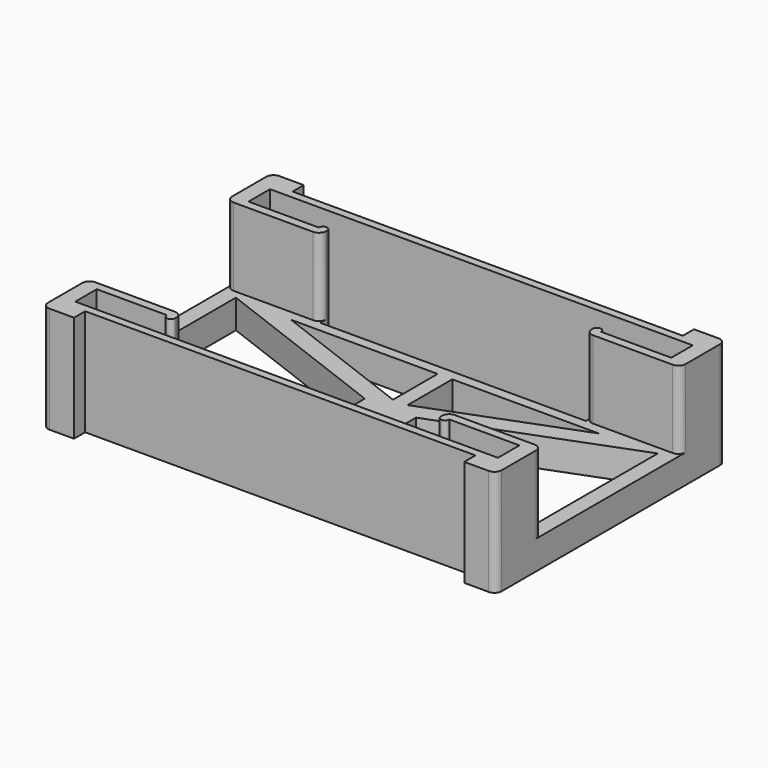
from build123d import *

# Parameters (mm, degrees)
F1_DEPTH = 7.4
F0_W     = 31.5
F0_H     = 12
F2_DEPTH = 2
F4_DEPTH = 25
F5_R     = 0.5
F6_R     = 0.5


# Not quite as in the source:
# - a feature names something its author has since deleted; it is built from what else it names


with BuildPart() as f1:
    # F0 (on Top) → F1 (new body)
    with BuildSketch(Plane.XY):
        Polygon((15.75, -9), (15.75, -6), (-15.75, -6), (-15.75, -9), (-15.75, -9.970754717), (-13.55, -9.970754717), (-13.55, -9), (13.55, -9), (13.55, -9.970754717), (15.75, -9.970754717), align=None)
    extrude(amount=F1_DEPTH)



with BuildPart() as f1b:
    # F0 (on Top) → F1, piece 2 (new body)
    with BuildSketch(Plane.XY):
        Polygon((13.55, 9.970754717), (13.55, 9), (-13.55, 9), (-13.55, 9.970754717), (-15.75, 9.970754717), (-15.75, 9), (-15.75, 6), (15.75, 6), (15.75, 9), (15.75, 9.970754717), align=None)
    extrude(amount=F1_DEPTH)


with BuildPart() as f1_1:
    add(f1.part)

    add(f1b.part)  # F2 merges F1b
    # F0 (on Top) → F2 (join)
    with BuildSketch(Plane.XY):
        Rectangle(F0_W, F0_H)
    extrude(amount=F2_DEPTH)

    # F3 (on face) → F4 (cut)
    with BuildSketch(Plane.XY):
        Polygon((-0.5079215625, -1.4132374693), (-10.6910164902, -5.2925117274), (-0.5079215625, -5.2925117274), align=None)
        Polygon((10.6910164902, -5.2925117274), (0.5079215625, -1.4132374693), (0.5079215625, -5.2925117274), align=None)
        Polygon((1.7789258686, -0.5523047257), (14.6478014067, -5.4547335021), (14.6478014067, -0.5523047257), (14.6478014067, 0.5523047257), (14.6478014067, 5.4547335021), (1.7789258686, 0.5523047257), align=None)
        Polygon((0.5079215625, 1.4132374693), (10.6910164902, 5.2925117274), (0.5079215625, 5.2925117274), align=None)
        Polygon((-0.5079215625, 5.2925117274), (-10.6910164902, 5.2925117274), (-0.5079215625, 1.4132374693), align=None)
        with BuildLine():
            Line((-9.222632274, 6), (9.222632274, 6))
            Line((9.222632274, 6), (9.222632274, 6.5901111811))
            ThreePointArc((9.222632274, 6.5901111811), (9.513632274, 6.8811111811), (9.804632274, 6.5901111811))
            Line((9.804632274, 6.5901111811), (13.0790583789, 6.5901111811))
            Line((13.0790583789, 6.5901111811), (13.7675590813, 6.5901111811))
            Line((13.7675590813, 6.5901111811), (14.6781420335, 6.5901111811))
            Line((14.6781420335, 6.5901111811), (14.6781420335, 8.4549048916))
            Line((14.6781420335, 8.4549048916), (13.7675590813, 8.4549048916))
            Line((13.7675590813, 8.4549048916), (13.0790583789, 8.4549048916))
            Line((13.0790583789, 8.4549048916), (7.4084047228, 8.4549048916))
            Line((7.4084047228, 8.4549048916), (6.8271243945, 8.4549048916))
            Line((6.8271243945, 8.4549048916), (-6.8271243945, 8.4549048916))
            Line((-6.8271243945, 8.4549048916), (-7.4084047228, 8.4549048916))
            Line((-7.4084047228, 8.4549048916), (-13.0790583789, 8.4549048916))
            Line((-13.0790583789, 8.4549048916), (-13.7675590813, 8.4549048916))
            Line((-13.7675590813, 8.4549048916), (-14.6781420335, 8.4549048916))
            Line((-14.6781420335, 8.4549048916), (-14.6781420335, 6.5901111811))
            Line((-14.6781420335, 6.5901111811), (-13.7675590813, 6.5901111811))
            Line((-13.7675590813, 6.5901111811), (-13.0790583789, 6.5901111811))
            Line((-13.0790583789, 6.5901111811), (-9.804632274, 6.5901111811))
            ThreePointArc((-9.804632274, 6.5901111811), (-9.513632274, 6.8811111811), (-9.222632274, 6.5901111811))
            Line((-9.222632274, 6.5901111811), (-9.222632274, 6))
        make_face()
        Polygon((-14.6478014067, 5.4547335021), (-14.6478014067, 0.5523047257), (-14.6478014067, -0.5523047257), (-14.6478014067, -5.4547335021), (-1.7789258686, -0.5523047257), (-1.7789258686, 0.5523047257), align=None)
        with BuildLine():
            Line((9.222632274, -6.5901111811), (9.222632274, -6))
            Line((9.222632274, -6), (-9.222632274, -6))
            Line((-9.222632274, -6), (-9.222632274, -6.5901111811))
            ThreePointArc((-9.222632274, -6.5901111811), (-9.513632274, -6.8811111811), (-9.804632274, -6.5901111811))
            Line((-9.804632274, -6.5901111811), (-13.0790583789, -6.5901111811))
            Line((-13.0790583789, -6.5901111811), (-13.7675590813, -6.5901111811))
            Line((-13.7675590813, -6.5901111811), (-14.6781420335, -6.5901111811))
            Line((-14.6781420335, -6.5901111811), (-14.6781420335, -8.4549048916))
            Line((-14.6781420335, -8.4549048916), (-13.7675590813, -8.4549048916))
            Line((-13.7675590813, -8.4549048916), (-13.0790583789, -8.4549048916))
            Line((-13.0790583789, -8.4549048916), (-7.4084047228, -8.4549048916))
            Line((-7.4084047228, -8.4549048916), (-6.8271243945, -8.4549048916))
            Line((-6.8271243945, -8.4549048916), (6.8271243945, -8.4549048916))
            Line((6.8271243945, -8.4549048916), (7.4084047228, -8.4549048916))
            Line((7.4084047228, -8.4549048916), (13.0790583789, -8.4549048916))
            Line((13.0790583789, -8.4549048916), (13.7675590813, -8.4549048916))
            Line((13.7675590813, -8.4549048916), (14.6781420335, -8.4549048916))
            Line((14.6781420335, -8.4549048916), (14.6781420335, -6.5901111811))
            Line((14.6781420335, -6.5901111811), (13.7675590813, -6.5901111811))
            Line((13.7675590813, -6.5901111811), (13.0790583789, -6.5901111811))
            Line((13.0790583789, -6.5901111811), (9.804632274, -6.5901111811))
            ThreePointArc((9.804632274, -6.5901111811), (9.513632274, -6.8811111811), (9.222632274, -6.5901111811))
        make_face()
    extrude(amount=F4_DEPTH, mode=Mode.SUBTRACT)

    # F5
    f5_edges = [f1_1.edges().sort_by_distance(p)[0] for p in [
        (-15.75, 6, 4.7),
        (-15.75, -6, 4.7),
        (15.75, 6, 4.7),
        (15.75, -6, 4.7),
        (15.75, -9.970755, 3.7),
        (-15.75, -9.970755, 3.7),
        (-15.75, 9.970755, 3.7),
        (15.75, 9.970755, 3.7),
    ]]
    fillet(f5_edges, radius=F5_R)

    # F6
    f6_edges = [f1_1.edges().sort_by_distance(p)[0] for p in [
        (-9.222632, 6, 4.7),
        (9.222632, 6, 4.7),
        (9.222632, -6, 4.7),
        (-9.222632, -6, 4.7),
    ]]
    fillet(f6_edges, radius=F6_R)


solid = f1_1.part
